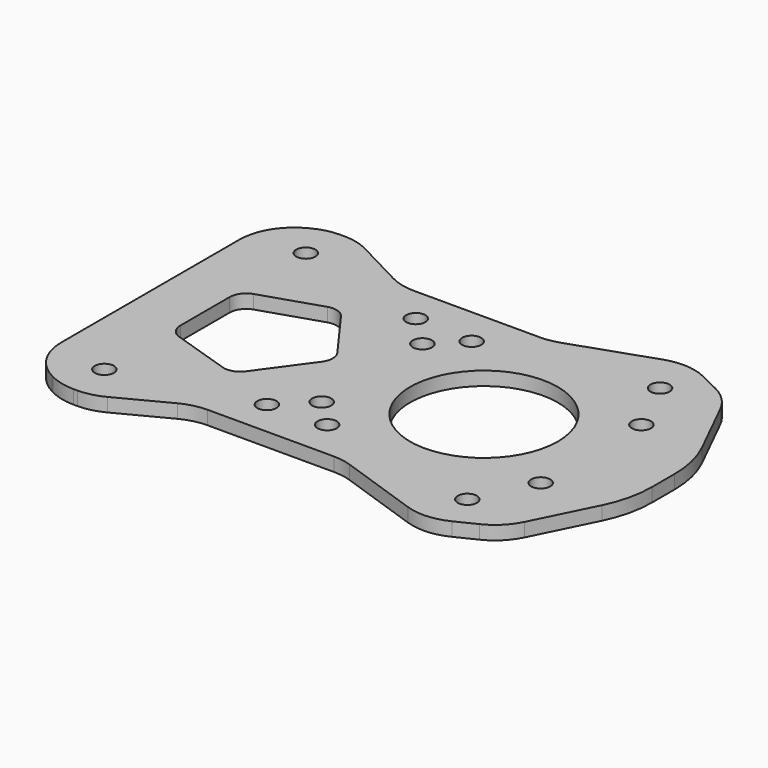
from build123d import *

# Parameters (mm, degrees)
F1_R     = 1.75
F1_R_2   = 13.5
F2_DEPTH = 2.5


with BuildPart() as f2:
    # F1 (on Top) → F2 (new body)
    with BuildSketch(Plane.XY):
        with BuildLine():
            Line((10.2372021925, 69.3784194525), (9.8985145849, 69.2028852716))
            ThreePointArc((9.8985145849, 69.2028852716), (5.955561629, 65.5199035219), (4.5, 60.324465819))
            Line((4.5, 60.324465819), (4.5, 40))
            Line((4.5, 40), (4.5, 19.675534181))
            ThreePointArc((4.5, 19.675534181), (5.955561629, 14.4800964781), (9.8985145849, 10.7971147284))
            Line((9.8985145849, 10.7971147284), (10.2372021925, 10.6215805475))
            ThreePointArc((10.2372021925, 10.6215805475), (12.470586525, 9.7844404555), (14.8386876076, 9.5))
            Line((14.8386876076, 9.5), (15.5546120462, 9.5))
            ThreePointArc((15.5546120462, 9.5), (17.9366290245, 9.7878429216), (20.1815166575, 10.634800977))
            Line((20.1815166575, 10.634800977), (29.1640234003, 15.322930568))
            ThreePointArc((29.1640234003, 15.322930568), (31.4089110333, 16.1698886233), (33.7909280117, 16.457731545))
            Line((33.7909280117, 16.457731545), (56.8851493299, 16.457731545))
            ThreePointArc((56.8851493299, 16.457731545), (58.5333421059, 16.3209693791), (60.1364527991, 15.9144236596))
            Line((60.1364527991, 15.9144236596), (74.8714324464, 10.8483931845))
            ThreePointArc((74.8714324464, 10.8483931845), (78.7421893122, 10.3242898655), (82.518433429, 11.3230007209))
            Line((82.518433429, 11.3230007209), (86.1698560542, 13.1099522035))
            ThreePointArc((86.1698560542, 13.1099522035), (88.830601645, 15.0063744472), (90.7380024689, 17.6592608982))
            Line((90.7380024689, 17.6592608982), (96.1243657197, 28.5514243616))
            ThreePointArc((96.1243657197, 28.5514243616), (97.6717100474, 32.8647106004), (98.1966778636, 37.4169761286))
            Line((98.1966778636, 37.4169761286), (98.1966778636, 40))
            Line((98.1966778636, 40), (98.1966778636, 42.5830238714))
            ThreePointArc((98.1966778636, 42.5830238714), (97.6717100474, 47.1352893996), (96.1243657197, 51.4485756384))
            Line((96.1243657197, 51.4485756384), (90.7380024689, 62.3407391018))
            ThreePointArc((90.7380024689, 62.3407391018), (88.830601645, 64.9936255528), (86.1698560542, 66.8900477965))
            Line((86.1698560542, 66.8900477965), (82.518433429, 68.6769992791))
            ThreePointArc((82.518433429, 68.6769992791), (78.7421893122, 69.6757101345), (74.8714324464, 69.1516068155))
            Line((74.8714324464, 69.1516068155), (60.1364527991, 64.0855763404))
            ThreePointArc((60.1364527991, 64.0855763404), (58.5333421059, 63.6790306209), (56.8851493299, 63.542268455))
            Line((56.8851493299, 63.542268455), (33.7909280117, 63.542268455))
            ThreePointArc((33.7909280117, 63.542268455), (31.4089110333, 63.8301113767), (29.1640234003, 64.677069432))
            Line((29.1640234003, 64.677069432), (20.1815166575, 69.365199023))
            ThreePointArc((20.1815166575, 69.365199023), (17.9366290245, 70.2121570784), (15.5546120462, 70.5))
            Line((15.5546120462, 70.5), (14.8386876076, 70.5))
            ThreePointArc((14.8386876076, 70.5), (12.470586525, 70.2155595445), (10.2372021925, 69.3784194525))
        make_face()
        with Locations((14.5, 17)):
            Circle(F1_R, mode=Mode.SUBTRACT)
        with Locations((39.3913947046, 23)):
            Circle(F1_R, mode=Mode.SUBTRACT)
        with Locations((50, 23.5)):
            Circle(F1_R, mode=Mode.SUBTRACT)
        with BuildLine():
            ThreePointArc((27.2737251007, 51.9557933746), (29.1278270669, 51.9557933746), (30.6278270669, 50.8659795825))
            Line((30.6278270669, 50.8659795825), (37.2412703927, 41.7633557569))
            ThreePointArc((37.2412703927, 41.7633557569), (37.8142194096, 40), (37.2412703927, 38.2366442431))
            Line((37.2412703927, 38.2366442431), (30.6278270669, 29.1340204175))
            ThreePointArc((30.6278270669, 29.1340204175), (29.1278270669, 28.0442066254), (27.2737251007, 28.0442066254))
            Line((27.2737251007, 28.0442066254), (16.5729490169, 31.52109954))
            ThreePointArc((16.5729490169, 31.52109954), (15.0729490169, 32.6109133321), (14.5, 34.3742690889))
            Line((14.5, 34.3742690889), (14.5, 45.6257309111))
            ThreePointArc((14.5, 45.6257309111), (15.0729490169, 47.3890866679), (16.5729490169, 48.47890046))
            Line((16.5729490169, 48.47890046), (27.2737251007, 51.9557933746))
        make_face(mode=Mode.SUBTRACT)
        with Locations((45, 28.5)):
            Circle(F1_R, mode=Mode.SUBTRACT)
        with Locations((80, 18)):
            Circle(F1_R, mode=Mode.SUBTRACT)
        with Locations((85, 28.5)):
            Circle(F1_R, mode=Mode.SUBTRACT)
        with Locations((45, 51.5)):
            Circle(F1_R, mode=Mode.SUBTRACT)
        with Locations((14.5, 63)):
            Circle(F1_R, mode=Mode.SUBTRACT)
        with Locations((39.3913947046, 57)):
            Circle(F1_R, mode=Mode.SUBTRACT)
        with Locations((50, 56.5)):
            Circle(F1_R, mode=Mode.SUBTRACT)
        with Locations((65.432921052, 40)):
            Circle(F1_R_2, mode=Mode.SUBTRACT)
        with Locations((85, 51.5)):
            Circle(F1_R, mode=Mode.SUBTRACT)
        with Locations((80, 62)):
            Circle(F1_R, mode=Mode.SUBTRACT)
    extrude(amount=F2_DEPTH)


solid = f2.part
